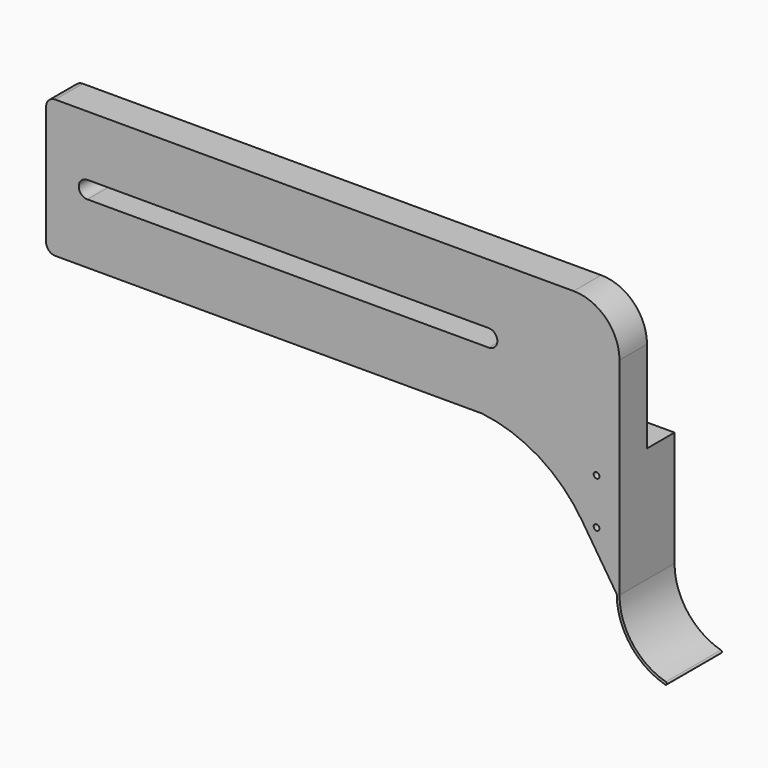
from build123d import *

# Parameters (mm, degrees)
F0_R           = 1.3992842893
F1_DEPTH       = 19.05
F2_R           = 5.08
F3_R           = 25.4
F4_R           = 1.3992842893
F5_DEPTH       = 19.05
F7_D           = 3.175
F7_CSINK_D     = 9.525
F7_CSINK_ANGLE = 90
F9_DEPTH       = 38.101
F11_DEPTH      = 19.05
F11_DEPTH_BACK = 19.05


with BuildPart() as f1:
    # F0 (on Front) → F1 (new body)
    with BuildSketch(Plane.XZ):
        with BuildLine():
            Line((150.8562757823, 76.2), (-166.6437242177, 76.2))
            Line((-166.6437242177, 76.2), (-166.6437242177, 0))
            Line((-166.6437242177, 0), (74.6562757823, 0))
            ThreePointArc((74.6562757823, 0), (106.2243540544, -10.8596763882), (130.1055285482, -34.187034615))
            Line((130.1055285482, -34.187034615), (150.8562757823, -66.1403832537))
            Line((150.8562757823, -66.1403832537), (150.8562757823, 76.2))
        make_face()
        with Locations((138.1562757823, -34.925)):
            Circle(F0_R, mode=Mode.SUBTRACT)
        with Locations((138.1562757823, -9.525)):
            Circle(F0_R, mode=Mode.SUBTRACT)
        with BuildLine():
            Line((78.4662757823, 33.3375), (-143.7837242177, 33.3375))
            ThreePointArc((-143.7837242177, 33.3375), (-148.5462242177, 38.1), (-143.7837242177, 42.8625))
            Line((-143.7837242177, 42.8625), (78.4662757823, 42.8625))
            ThreePointArc((78.4662757823, 42.8625), (83.2287757823, 38.1), (78.4662757823, 33.3375))
        make_face(mode=Mode.SUBTRACT)
        with Locations((138.1562757823, -34.925)):
            Circle(F0_R)
        with Locations((138.1562757823, -9.525)):
            Circle(F0_R)
    extrude(amount=F1_DEPTH)

    # F2
    f2_edges = [f1.edges().sort_by_distance(p)[0] for p in [
        (-166.643724, -9.525, 76.2),
        (-166.643724, -9.525, 0),
    ]]
    fillet(f2_edges, radius=F2_R)

    # F3
    f3_edges = [f1.edges().sort_by_distance(p)[0] for p in [
        (150.856276, -9.525, 76.2),
    ]]
    fillet(f3_edges, radius=F3_R)

    # F4 (on face) → F5 (join)
    with BuildSketch(Plane(origin=(0, 0, 0), x_dir=(-1, 0, 0), z_dir=(0, 1, 0))):
        with BuildLine():
            Line((-150.8562757823, 0), (-150.8562757823, -66.1403832537))
            Line((-150.8562757823, -66.1403832537), (-130.1055285482, -34.187034615))
            ThreePointArc((-130.1055285482, -34.187034615), (-106.2243540544, -10.8596763882), (-74.6562757823, 0))
            Line((-74.6562757823, 0), (-150.8562757823, 0))
        make_face()
        with Locations((-138.1562757823, -34.925)):
            Circle(F4_R, mode=Mode.SUBTRACT)
        with Locations((-138.1562757823, -9.525)):
            Circle(F4_R, mode=Mode.SUBTRACT)
        with Locations((-138.1562757823, -34.925)):
            Circle(F4_R)
        with Locations((-138.1562757823, -9.525)):
            Circle(F4_R)
    extrude(amount=F5_DEPTH)

    # F7 (through all)
    with Locations(Plane(origin=(0, 19.05, 0), x_dir=(-1, 0, 0), z_dir=(0, 1, 0))):
        with Locations((-138.1562757823, -34.925), (-138.1562757823, -9.525)):
            CounterSinkHole(F7_D / 2, F7_CSINK_D / 2, counter_sink_angle=F7_CSINK_ANGLE)

    # F8 (on face) → F9 (cut, through all)
    with BuildSketch(Plane.XZ.offset(19.05)):
        Polygon((150.8562757823, -66.1403832537), (150.8562757823, -2.6403832537), (149.3322757823, -2.6403832537), (149.3322757823, -63.7936290488), align=None)
    extrude(amount=-F9_DEPTH, mode=Mode.SUBTRACT)

    # F10 (on Front) → F11 (join, two sides)
    with BuildSketch(Plane.XZ) as f11_sk:
        with BuildLine():
            Line((150.8562757823, -63.7936290488), (150.8562757823, -2.6403832537))
            Line((150.8562757823, -2.6403832537), (149.3322757823, -2.6403832537))
            Line((149.3322757823, -2.6403832537), (149.3322757823, -63.7936290488))
            ThreePointArc((149.3322757823, -63.7936290488), (156.7895472638, -85.9779592892), (176.1329621077, -99.1532281041))
            ThreePointArc((176.1329621077, -99.1532281041), (177.0725432504, -98.6255205372), (176.5448356835, -97.6859393944))
            ThreePointArc((176.5448356835, -97.6859393944), (158.004098895, -85.0573940633), (150.8562757823, -63.7936290488))
        make_face()
    extrude(amount=F11_DEPTH)
    extrude(f11_sk.sketch, amount=-F11_DEPTH_BACK)


solid = f1.part
